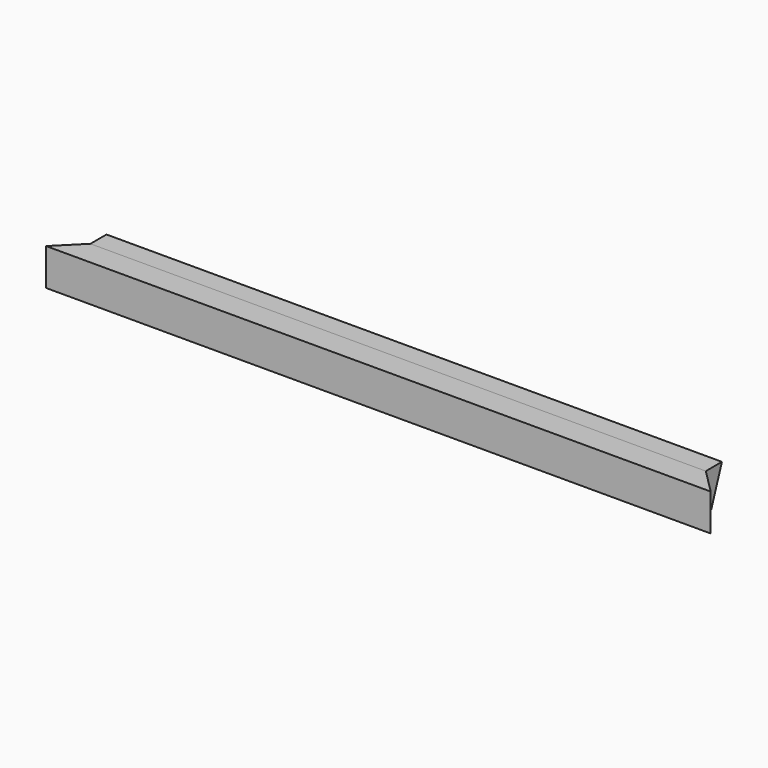
from build123d import *

# Parameters (mm, degrees)
F0_W        = 270
F0_H        = 15
F1_DEPTH    = 10
F2_SIZE     = 9.99999
F3_W        = 250.00002
F3_H        = 15
F4_DEPTH    = 10
F5_T1_DEPTH = 353.767809302


# Not quite as in the source:
# - a fillet or chamfer that OpenCascade refuses, or shapes differently, is made with other operations: its cross-section is extruded or revolved along the edge and cut away or added
# - a fillet or chamfer is up to 0.001 mm smaller than in the source, because OpenCascade refuses the exact size
# - a feature of the source that left no trace in its solid (it failed there, or was rolled back) is left out


with BuildPart() as f1:
    # F0 (on Front) → F1 (new body)
    with BuildSketch(Plane.XZ):
        Rectangle(F0_W, F0_H)
    extrude(amount=F1_DEPTH)

    # F2 (size 10 in the source; OpenCascade refuses exactly that, so slightly less here)
    f2_edges = [f1.edges().sort_by_distance(p)[0] for p in [
        (135, 0, 0),
        (-135, 0, 0),
    ]]
    chamfer(f2_edges, length=F2_SIZE)


with BuildPart() as f4:
    # F3 (on face) → F4 (new body)
    with BuildSketch(Plane(origin=(0, 0, 0), x_dir=(-1, 0, 0), z_dir=(0, 1, 0))):
        Rectangle(F3_W, F3_H)
    extrude(amount=F4_DEPTH)

    # F5: chamfer of 20 x 7.2794046853 on 1 edges, made by hand

    # F5_s2 → F5_t1 (cut)
    with BuildSketch(Plane.YZ.offset(-176.883904651)):
        Polygon((2.7205953147, -7.5), (10, 12.5), (10, -7.5), align=None)
    extrude(amount=F5_T1_DEPTH, mode=Mode.SUBTRACT)


solid = Compound([f1.part, f4.part])
